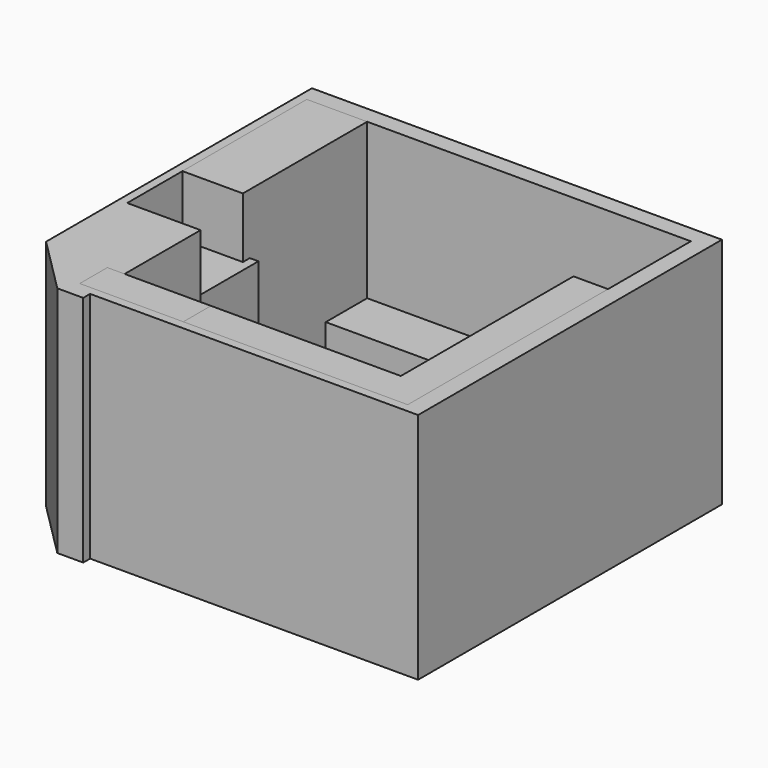
from build123d import *

# Parameters (mm, degrees)
F1_DEPTH       = 2700
F2_W           = 700
F2_H           = 2700
F3_DEPTH       = 1800
F4_W           = 500
F4_H           = 400
F5_DEPTH       = 750
F6_W           = 600
F6_H           = 900
F7_DEPTH       = 1200
F9_DEPTH       = 2900
F11_DEPTH      = 2000
F11_DEPTH_BACK = 200
F13_DEPTH      = 1200
F14_W          = 3850
F14_H          = 600
F15_DEPTH      = 900
F14_W_2        = 800
F14_H_2        = 900
F16_DEPTH      = 2000


with BuildPart() as f1:
    # F0 (on Top) → F1 (new body)
    with BuildSketch(Plane.XY):
        Polygon((-1375, -2658.0309391022), (-1375, -2558.0309391022), (2425, -2558.0309391022), (2425, 1841.9690608978), (-2325, 1841.9690608978), (-2325, -2008.0309391022), (-1675, -2658.0309391022), align=None)
        Polygon((-2225, -958.0309391022), (-2225, 1641.9690608978), (2225, 1641.9690608978), (2225, -2458.0309391022), (-1375, -2458.0309391022), (-1375, -958.0309391022), align=None, mode=Mode.SUBTRACT)
    extrude(amount=F1_DEPTH)


with BuildPart() as f3:
    # F2 (on face) → F3 (new body)
    with BuildSketch(Plane.XZ.offset(-1641.9690608978)):
        with Locations((-1875, 1350)):
            Rectangle(F2_W, F2_H)
    extrude(amount=F3_DEPTH)


with BuildPart() as f5:
    # F4 (on Top) → F5 (new body)
    with BuildSketch(Plane.XY):
        with Locations((-325, -50)):
            Rectangle(F4_W, F4_H)
        Polygon((825, 300), (-75, 300), (-75, 150), (-75, -250), (-75, -400), (825, -400), (825, -250), (825, 150), align=None)
        with Locations((1075, -50)):
            Rectangle(F4_W, F4_H)
        Polygon((825, -400), (-75, -400), (-75, -550), (-75, -950), (-75, -1100), (825, -1100), (825, -950), (825, -550), align=None)
        with Locations((-325, -750)):
            Rectangle(F4_W, F4_H)
        with Locations((1075, -750)):
            Rectangle(F4_W, F4_H)
    extrude(amount=F5_DEPTH)


with BuildPart() as f7:
    # F6 (on face) → F7 (new body)
    with BuildSketch(Plane.XZ.offset(-1641.9690608978)):
        with Locations((1925, 450)):
            Rectangle(F6_W, F6_H)
    extrude(amount=F7_DEPTH)


with BuildPart() as f9:
    # F8 (on face) → F9 (new body, through all)
    with BuildSketch(Plane.XZ.offset(-441.9690608978)):
        Polygon((2215, 900), (2225, 900), (2225, 2700), (1825, 2700), (1825, 1500), (2215, 1500), align=None)
        Polygon((1625, 0), (2225, 0), (2225, 900), (2215, 900), (1625, 900), align=None)
    extrude(amount=F9_DEPTH)

    # F10 (on face) → F11 (join, two sides)
    with BuildSketch(Plane(origin=(1625, 0, 0), x_dir=(0, -1, 0), z_dir=(-1, 0, 0))) as f11_sk:
        Polygon((2448.0309391022, 900), (2458.0309391022, 900), (2458.0309391022, 2700), (2058.0309391022, 2700), (2058.0309391022, 1500), (2448.0309391022, 1500), align=None)
        Polygon((2058.0309391022, 0), (2458.0309391022, 0), (2458.0309391022, 900), (2448.0309391022, 900), (2058.0309391022, 900), align=None)
    extrude(amount=F11_DEPTH)
    extrude(f11_sk.sketch, amount=-F11_DEPTH_BACK)


with BuildPart() as f13:
    # F12 (on face) → F13 (new body)
    with BuildSketch(Plane(origin=(-375, 0, 0), x_dir=(0, -1, 0), z_dir=(-1, 0, 0))):
        Polygon((2458.0309391022, 0), (2458.0309391022, 2700), (2058.0309391022, 2700), (2058.0309391022, 1500), (2448.0309391022, 1500), (2448.0309391022, 900), (2058.0309391022, 900), (2058.0309391022, 0), align=None)
    extrude(amount=F13_DEPTH)


with BuildPart() as f15:
    # F14 (on Top) → F15 (new body)
    with BuildSketch(Plane.XY):
        with Locations((-300, 1341.9690608978)):
            Rectangle(F14_W, F14_H)
    extrude(amount=F15_DEPTH)


with BuildPart() as f16:
    # F14 (on Top) → F16 (new body)
    with BuildSketch(Plane.XY):
        with Locations((-1825, -508.0309391022)):
            Rectangle(F14_W_2, F14_H_2)
    extrude(amount=F16_DEPTH)


solid = Compound([f1.part, f3.part, f5.part, f7.part, f9.part, f13.part, f15.part, f16.part])
